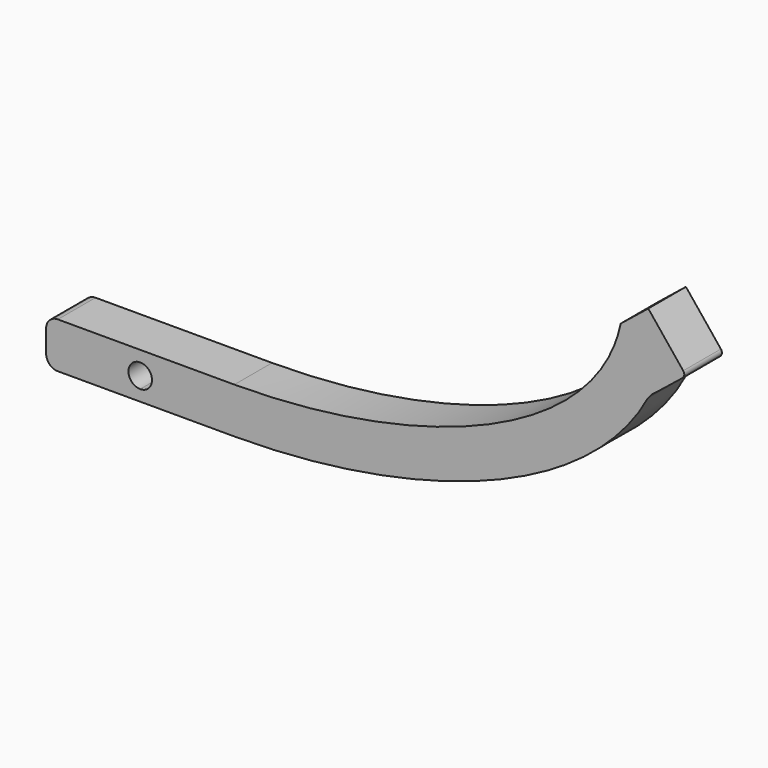
from build123d import *

# Parameters (mm, degrees)
F1_DEPTH = 10


# Not quite as in the source:
# - ends of sketch curves that miss each other by under 0.0002 mm in the source are joined
# - the dataset's text gives a spline's control points without its knots; the knots are read off the source's solid


with BuildPart() as f1:
    # F0 (on Front) → F1 (new body)
    with BuildSketch(Plane.XZ):
        with BuildLine():
            Line((-65.2858525045, 19.1747198819), (-82.7858525045, 19.1747198819))
            ThreePointArc((-82.7858525045, 19.1747198819), (-84.5536194575, 18.4424868349), (-85.2858525045, 16.6747198819))
            Line((-85.2858525045, 16.6747198819), (-85.2858525045, 11.9747207331))
            ThreePointArc((-85.2858525045, 11.9747207331), (-84.5536194575, 10.2069537801), (-82.7858525045, 9.4747207331))
            Line((-82.7858525045, 9.4747207331), (-65.2858525045, 9.4747207331))
            Line((-65.2858525045, 9.4747207331), (-65.2858525045, 11.8247203075))
            ThreePointArc((-65.2858525045, 11.8247203075), (-67.7858525045, 14.3247203075), (-65.2858525045, 16.8247203075))
            Line((-65.2858525045, 16.8247203075), (-65.2858525045, 19.1747198819))
        make_face()
        with BuildLine():
            Line((-45.2858542078, 19.1747198819), (-65.2858525045, 19.1747198819))
            Line((-65.2858525045, 19.1747198819), (-65.2858525045, 16.8247203075))
            ThreePointArc((-65.2858525045, 16.8247203075), (-63.5180855515, 16.0924872605), (-62.7858525045, 14.3247203075))
            ThreePointArc((-62.7858525045, 14.3247203075), (-63.5180855515, 12.5569533545), (-65.2858525045, 11.8247203075))
            Line((-65.2858525045, 11.8247203075), (-65.2858525045, 9.4747207331))
            Line((-65.2858525045, 9.4747207331), (-45.2858525045, 9.4747207331))
            Line((-45.2858525045, 9.4747207331), (-45.2858542078, 19.1747198819))
        make_face()
        with BuildLine():
            add(Edge.make_bspline(
                [(-45.2858542078, 19.1747198819), (-7.4020708747, 19.1747265342), (31.6102094948, 32.6948724687), (36.8064381182, 57.2929121554)],
                knots=[0, 0, 0, 0, 90.5104471403, 90.5104471403, 90.5104471403, 90.5104471403], degree=3))
            Line((-45.2858542078, 19.1747198819), (-45.2858525045, 9.4747207331))
            add(Edge.make_bspline(
                [(-45.2858525045, 9.4747207331), (-40.2618978901, 9.4747216153), (-30.1894784684, 9.9223917761), (-15.362918013, 11.9100905112), (-1.1709415961, 15.2094571968), (12.0418148644, 19.8491680066), (21.9570020274, 24.9039048155), (29.047465051, 29.7583646646), (33.8850587667, 33.8431124408), (38.1663250739, 38.413322434), (40.9420261226, 42.3174471625), (42.2861221075, 44.6734195955), (42.5837097689, 45.2249895308)],
                knots=[0, 0, 0, 0, 0.125, 0.25, 0.375, 0.5, 0.625, 0.6875, 0.75, 0.8125, 0.875, 0.8937572345, 0.8937572345, 0.8937572345, 0.8937572345], degree=3))
            add(Edge.make_bspline(
                [(42.5837097689, 45.2249895308), (42.9712246909, 45.9432369861), (43.3372375793, 46.6745796576), (43.6802036603, 47.4185139687)],
                knots=[0.8937572345, 0.8937572345, 0.8937572345, 0.8937572345, 0.9181826701, 0.9181826701, 0.9181826701, 0.9181826701], degree=3))
            Line((43.6802036603, 47.4185139687), (44.295853648, 46.8606554446))
            Line((44.295853648, 46.8606554446), (49.9209338751, 51.373229087))
            ThreePointArc((49.9209338751, 51.373229087), (50.2893303324, 52.0452304101), (50.0738615656, 52.7806724123))
            Line((50.0738615656, 52.7806724123), (42.6465372943, 61.9985727481))
            Line((42.6465372943, 61.9985727481), (36.8064381182, 57.2929121554))
        make_face()
        with BuildLine():
            add(Edge.make_bspline(
                [(42.5837097689, 45.2249895308), (42.9712246909, 45.9432369861), (43.3372375793, 46.6745796576), (43.6802036603, 47.4185139687)],
                knots=[0.8937572345, 0.8937572345, 0.8937572345, 0.8937572345, 0.9181826701, 0.9181826701, 0.9181826701, 0.9181826701], degree=3))
            add(Edge.make_bspline(
                [(42.5837097689, 45.2249895308), (42.9444412623, 45.4831122336), (42.9444412623, 45.9540075538), (44.295853648, 46.8606554446)],
                knots=[0, 0, 0, 0, 2.3678540998, 2.3678540998, 2.3678540998, 2.3678540998], degree=3))
            Line((44.295853648, 46.8606554446), (43.6802036603, 47.4185139687))
        make_face()
    extrude(amount=F1_DEPTH)


solid = f1.part
